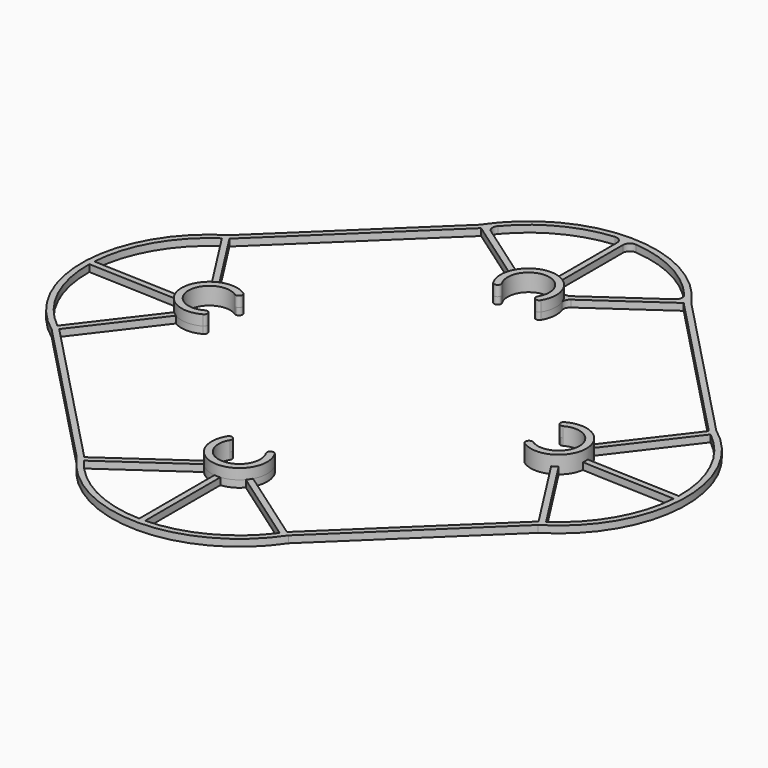
from build123d import *

# Parameters (mm, degrees)
F1_DEPTH = 2
F2_R     = 0.99999
F3_R     = 2
F6_DEPTH = 3


# Not quite as in the source:
# - a fillet or chamfer is up to 0.001 mm smaller than in the source, because OpenCascade refuses the exact size


with BuildPart() as f1:
    # F0 (on Top) → F1 (new body)
    with BuildSketch(Plane.XY):
        with BuildLine():
            Line((73.5948921635, -24.4738152558), (30.4890723007, 20.4280804346))
            ThreePointArc((30.4890723007, 20.4280804346), (0, 36.7), (-30.4890723007, 20.4280804346))
            Line((-30.4890723007, 20.4280804346), (-71.107024482, -18.5651536595))
            ThreePointArc((-71.107024482, -18.5651536595), (-88.6093292458, -48.364956076), (-73.5948921635, -79.4925254511))
            Line((-73.5948921635, -79.4925254511), (-30.4890723007, -124.3944211415))
            ThreePointArc((-30.4890723007, -124.3944211415), (0, -140.666340707), (30.4890723007, -124.3944211415))
            Line((30.4890723007, -124.3944211415), (71.107024482, -85.4011870475))
            ThreePointArc((71.107024482, -85.4011870475), (88.6093292458, -55.601384631), (73.5948921635, -24.4738152558))
        make_face()
        with BuildLine():
            Line((-28.1743255129, -124.7318742155), (-6.0285815603, -109.2252573607))
            ThreePointArc((-6.0285815603, -109.2252573607), (-3.6939889059, -111.0624273724), (-0.85, -111.9210562896))
            Line((-0.85, -111.9210562896), (-0.85, -138.9560177561))
            ThreePointArc((-0.85, -138.9560177561), (-16.1612014632, -135.0117198682), (-28.1743255129, -124.7318742155))
        make_face(mode=Mode.SUBTRACT)
        with BuildLine():
            ThreePointArc((-59.9226587205, -50.3870367891), (-59.1807775846, -53.2636891654), (-57.4403870983, -55.6712932586))
            Line((-57.4403870983, -55.6712932586), (-73.8376241337, -77.1659381522))
            ThreePointArc((-73.8376241337, -77.1659381522), (-83.618782922, -64.7434058486), (-86.9351098111, -49.2840283695))
            Line((-86.9351098111, -49.2840283695), (-59.9226587205, -50.3870367891))
        make_face(mode=Mode.SUBTRACT)
        with BuildLine():
            ThreePointArc((-5, -3.3166247904), (0, 6), (5, -3.3166247904))
            Line((5, -3.3166247904), (5, -6.2449979984))
            ThreePointArc((5, -6.2449979984), (7.847410611, -1.555039132), (7.0036615021, 3.8663581784))
            Line((7.0036615021, 3.8663581784), (29.1494054547, 19.3729750332))
            Line((29.1494054547, 19.3729750332), (72.4860077697, -25.7693190449))
            Line((72.4860077697, -25.7693190449), (56.0887707343, -47.2639639384))
            ThreePointArc((56.0887707343, -47.2639639384), (50.7063118949, -46.1997279693), (45.9040856171, -48.8534205162))
            Line((45.9040856171, -48.8534205162), (48.830020546, -48.9728961925))
            ThreePointArc((48.830020546, -48.9728961925), (57.9348912774, -54.3488450807), (48.4220272071, -58.9645697978))
            Line((48.4220272071, -58.9645697978), (45.4960922782, -58.8450941215))
            ThreePointArc((45.4960922782, -58.8450941215), (50.0659736435, -61.8814810638), (55.5172812862, -61.2596238927))
            Line((55.5172812862, -61.2596238927), (70.1074551181, -84.0195880634))
            Line((70.1074551181, -84.0195880634), (29.1494054547, -123.3393157402))
            Line((29.1494054547, -123.3393157402), (7.0036615021, -107.8326988854))
            ThreePointArc((7.0036615021, -107.8326988854), (7.847410611, -102.411301575), (5, -97.7213427086))
            Line((5, -97.7213427086), (5, -100.6497159166))
            ThreePointArc((5, -100.6497159166), (0, -109.966340707), (-5, -100.6497159166))
            Line((-5, -100.6497159166), (-5, -97.7213427086))
            ThreePointArc((-5, -97.7213427086), (-7.847410611, -102.411301575), (-7.0036615021, -107.8326988854))
            Line((-7.0036615021, -107.8326988854), (-29.1494054547, -123.3393157402))
            Line((-29.1494054547, -123.3393157402), (-72.4860077697, -78.1970216621))
            Line((-72.4860077697, -78.1970216621), (-56.0887707343, -56.7023767685))
            ThreePointArc((-56.0887707343, -56.7023767685), (-50.7063118949, -57.7666127376), (-45.9040856171, -55.1129201908))
            Line((-45.9040856171, -55.1129201908), (-48.830020546, -54.9934445145))
            ThreePointArc((-48.830020546, -54.9934445145), (-57.9348912774, -49.6174956263), (-48.4220272071, -45.0017709092))
            Line((-48.4220272071, -45.0017709092), (-45.4960922782, -45.1212465855))
            ThreePointArc((-45.4960922782, -45.1212465855), (-50.0659736435, -42.0848596432), (-55.5172812862, -42.7067168143))
            Line((-55.5172812862, -42.7067168143), (-70.1074551181, -19.9467526436))
            Line((-70.1074551181, -19.9467526436), (-29.1494054547, 19.3729750332))
            Line((-29.1494054547, 19.3729750332), (-7.0036615021, 3.8663581784))
            ThreePointArc((-7.0036615021, 3.8663581784), (-7.847410611, -1.555039132), (-5, -6.2449979984))
            Line((-5, -6.2449979984), (-5, -3.3166247904))
        make_face(mode=Mode.SUBTRACT)
        with BuildLine():
            Line((0.85, -138.9560177561), (0.85, -111.9210562896))
            ThreePointArc((0.85, -111.9210562896), (3.6939889059, -111.0624273724), (6.0285815603, -109.2252573607))
            Line((6.0285815603, -109.2252573607), (28.1743255129, -124.7318742155))
            ThreePointArc((28.1743255129, -124.7318742155), (16.1612014632, -135.0117198682), (0.85, -138.9560177561))
        make_face(mode=Mode.SUBTRACT)
        with BuildLine():
            ThreePointArc((56.9484628744, -60.3421712992), (58.8793530111, -58.0844778314), (59.8532998529, -55.2778884308))
            Line((59.8532998529, -55.2778884308), (86.8657509435, -56.3808968503))
            ThreePointArc((86.8657509435, -56.3808968503), (82.300050413, -71.5184248765), (71.5386367063, -83.1021354698))
            Line((71.5386367063, -83.1021354698), (56.9484628744, -60.3421712992))
        make_face(mode=Mode.SUBTRACT)
        with BuildLine():
            ThreePointArc((-56.9484628744, -43.6241694078), (-58.8793530111, -45.8818628756), (-59.8532998529, -48.6884522762))
            Line((-59.8532998529, -48.6884522762), (-86.8657509435, -47.5854438566))
            ThreePointArc((-86.8657509435, -47.5854438566), (-82.300050413, -32.4479158305), (-71.5386367063, -20.8642052372))
            Line((-71.5386367063, -20.8642052372), (-56.9484628744, -43.6241694078))
        make_face(mode=Mode.SUBTRACT)
        with BuildLine():
            ThreePointArc((-0.85, 7.9547155826), (-3.6939889059, 7.0960866654), (-6.0285815603, 5.2589166537))
            Line((-6.0285815603, 5.2589166537), (-28.1743255129, 20.7655335085))
            ThreePointArc((-28.1743255129, 20.7655335085), (-16.1612014632, 31.0453791612), (-0.85, 34.9896770491))
            Line((-0.85, 34.9896770491), (-0.85, 7.9547155826))
        make_face(mode=Mode.SUBTRACT)
        with BuildLine():
            ThreePointArc((59.9226587205, -53.5793039179), (59.1807775846, -50.7026515416), (57.4403870983, -48.2950474484))
            Line((57.4403870983, -48.2950474484), (73.8376241337, -26.8004025548))
            ThreePointArc((73.8376241337, -26.8004025548), (83.618782922, -39.2229348584), (86.9351098111, -54.6823123374))
            Line((86.9351098111, -54.6823123374), (59.9226587205, -53.5793039179))
        make_face(mode=Mode.SUBTRACT)
        with BuildLine():
            ThreePointArc((0.85, 34.9896770491), (16.1612014632, 31.0453791612), (28.1743255129, 20.7655335085))
            Line((28.1743255129, 20.7655335085), (6.0285815603, 5.2589166537))
            ThreePointArc((6.0285815603, 5.2589166537), (3.6939889059, 7.0960866654), (0.85, 7.9547155826))
            Line((0.85, 7.9547155826), (0.85, 34.9896770491))
        make_face(mode=Mode.SUBTRACT)
    extrude(amount=F1_DEPTH)

    # F2 (radius 1 in the source; OpenCascade refuses exactly that, so slightly less here)
    f2_edges = [f1.edges().sort_by_distance(p)[0] for p in [
        (-5, -3.316625, 1),
        (-5, -6.244998, 1),
        (5, -3.316625, 1),
        (5, -6.244998, 1),
        (48.830021, -48.972896, 1),
        (45.904086, -48.853421, 1),
        (48.422027, -58.96457, 1),
        (45.496092, -58.845094, 1),
        (5, -100.649716, 1),
        (5, -97.721343, 1),
        (-5, -97.721343, 1),
        (-5, -100.649716, 1),
        (-48.830021, -54.993445, 1),
        (-45.904086, -55.11292, 1),
        (-48.422027, -45.001771, 1),
        (-45.496092, -45.121247, 1),
    ]]
    fillet(f2_edges, radius=F2_R)

    # F3
    f3_edges = [f1.edges().sort_by_distance(p)[0] for p in [
        (6.028582, 5.258917, 1),
        (0.85, 7.954716, 1),
        (7.003662, 3.866358, 1),
        (-0.85, 7.954716, 1),
        (-7.003662, 3.866358, 1),
        (-6.028582, 5.258917, 1),
        (28.174326, 20.765534, 1),
        (-28.174326, 20.765534, 1),
        (-0.85, 34.989677, 1),
        (0.85, 34.989677, 1),
    ]]
    fillet(f3_edges, radius=F3_R)

    # F5 (on face) → F6 (join)
    with BuildSketch(Plane.XY.offset(2)):
        with BuildLine():
            ThreePointArc((-49.0618129875, -55.126955847), (-57.9348912774, -49.6174956263), (-48.6421626961, -44.8498058529))
            ThreePointArc((-48.6421626961, -44.8498058529), (-47.2571276636, -44.5640122932), (-47.5429212234, -43.1789772607))
            ThreePointArc((-47.5429212234, -43.1789772607), (-59.9332259985, -49.5358969586), (-48.1024549453, -56.8818439194))
            ThreePointArc((-48.1024549453, -56.8818439194), (-47.7046899302, -55.5247208621), (-49.0618129875, -55.126955847))
        make_face()
        with BuildLine():
            ThreePointArc((-6.8571428571, -99.8457106779), (0, -111.966340707), (6.8571428571, -99.8457106779))
            ThreePointArc((6.8571428571, -99.8457106779), (5.4849212464, -99.5036465744), (5.1428571429, -100.8758681852))
            ThreePointArc((5.1428571429, -100.8758681852), (0, -109.966340707), (-5.1428571429, -100.8758681852))
            ThreePointArc((-5.1428571429, -100.8758681852), (-5.4849212464, -99.5036465744), (-6.8571428571, -99.8457106779))
        make_face()
        with BuildLine():
            ThreePointArc((49.0618129875, -48.83938486), (57.9348912774, -54.3488450807), (48.6421626961, -59.1165348541))
            ThreePointArc((48.6421626961, -59.1165348541), (47.2571276636, -59.4023284138), (47.5429212234, -60.7873634463))
            ThreePointArc((47.5429212234, -60.7873634463), (59.9332259985, -54.4304437484), (48.1024549453, -47.0844967876))
            ThreePointArc((48.1024549453, -47.0844967876), (47.7046899302, -48.4416198449), (49.0618129875, -48.83938486))
        make_face()
        with BuildLine():
            ThreePointArc((-5.1428571429, -3.0904725218), (0, 6), (5.1428571429, -3.0904725218))
            ThreePointArc((5.1428571429, -3.0904725218), (5.4849212464, -4.4626941326), (6.8571428571, -4.1206300291))
            ThreePointArc((6.8571428571, -4.1206300291), (0, 8), (-6.8571428571, -4.1206300291))
            ThreePointArc((-6.8571428571, -4.1206300291), (-5.4849212464, -4.4626941326), (-5.1428571429, -3.0904725218))
        make_face()
    extrude(amount=F6_DEPTH)


solid = f1.part
